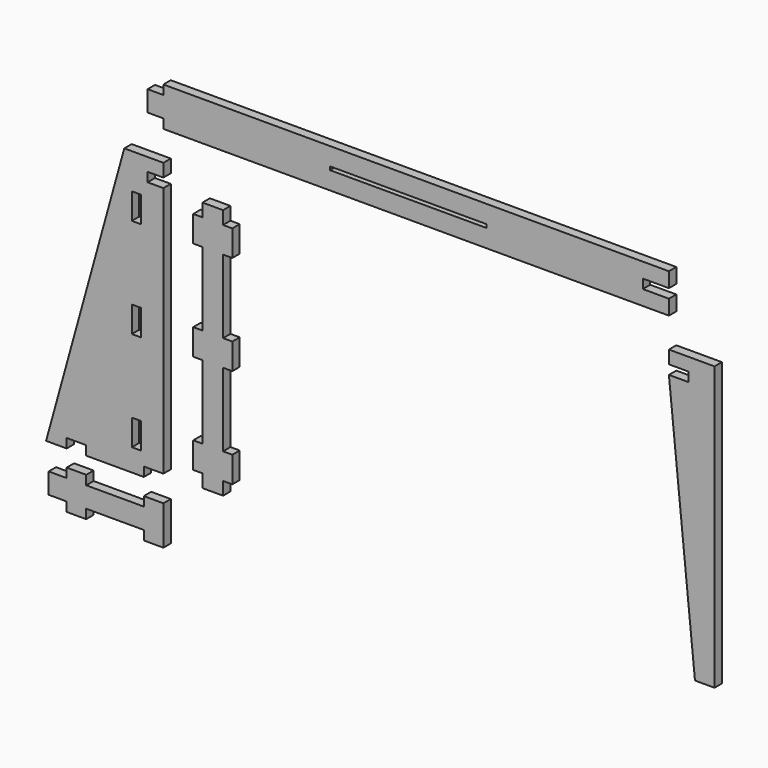
from build123d import *

# Parameters (mm, degrees)
F1_W     = 304.8
F1_H     = 6.604
F2_DEPTH = 18.034
F1_W_2   = 18.034
F1_H_2   = 50.8
F1_W_3   = 38.1
F1_H_3   = 18.034


# Not quite as in the source:
# - a variable given as a bare number and used for a length is read in inches; the dataset says mm whatever the document's units were


with BuildPart() as f2:
    # F1 (on Front) → F2 (new body)
    with BuildSketch(Plane.XZ):
        Polygon((508, 0), (-477.266, 0), (-477.266, -18.034), (-508, -18.034), (-508, -58.166), (-477.266, -58.166), (-477.266, -76.2), (508, -76.2), (508, -47.117), (457.2, -47.117), (457.2, -29.083), (508, -29.083), align=None)
        with Locations((0, -38.1)):
            Rectangle(F1_W, F1_H, mode=Mode.SUBTRACT)
    extrude(amount=F2_DEPTH)


with BuildPart() as f2b:
    # F1 (on Front) → F2, piece 2 (new body)
    with BuildSketch(Plane.XZ):
        Polygon((596.9, -685.8), (596.9, -134.366), (508, -134.366), (508, -159.766), (546.1, -159.766), (546.1, -177.8), (508, -177.8), (558.8, -685.8), align=None)
    extrude(amount=F2_DEPTH)


with BuildPart() as f2c:
    # F1 (on Front) → F2, piece 3 (new body)
    with BuildSketch(Plane.XZ):
        Polygon((-477.266, -667.766), (-477.266, -177.8), (-508, -177.8), (-508, -159.766), (-477.266, -159.766), (-477.266, -134.366), (-553.466, -134.366), (-705.866, -685.8), (-665.734, -685.8), (-665.734, -667.766), (-627.634, -667.766), (-627.634, -685.8), (-515.366, -685.8), (-515.366, -667.766), align=None)
        with Locations((-529.717, -616.966)):
            Rectangle(F1_W_2, F1_H_2, mode=Mode.SUBTRACT)
        with Locations((-529.717, -422.783)):
            Rectangle(F1_W_2, F1_H_2, mode=Mode.SUBTRACT)
        with Locations((-529.717, -228.6)):
            Rectangle(F1_W_2, F1_H_2, mode=Mode.SUBTRACT)
    extrude(amount=F2_DEPTH)


with BuildPart() as f2d:
    # F1 (on Front) → F2, piece 4 (new body)
    with BuildSketch(Plane.XZ):
        with Locations((-410.083, -228.6)):
            Rectangle(F1_W_2, F1_H_2)
        with Locations((-351.917, -228.6)):
            Rectangle(F1_W_2, F1_H_2)
        with Locations((-351.917, -422.783)):
            Rectangle(F1_W_2, F1_H_2)
        with Locations((-410.083, -422.783)):
            Rectangle(F1_W_2, F1_H_2)
        with Locations((-410.083, -616.966)):
            Rectangle(F1_W_2, F1_H_2)
        with Locations((-351.917, -616.966)):
            Rectangle(F1_W_2, F1_H_2)
        Polygon((-360.934, -177.8), (-401.066, -177.8), (-401.066, -203.2), (-401.066, -254), (-401.066, -397.383), (-401.066, -448.183), (-401.066, -591.566), (-401.066, -642.366), (-401.066, -667.766), (-360.934, -667.766), (-360.934, -642.366), (-360.934, -591.566), (-360.934, -448.183), (-360.934, -397.383), (-360.934, -254), (-360.934, -203.2), align=None)
    extrude(amount=F2_DEPTH)


with BuildPart() as f2e:
    # F1 (on Front) → F2, piece 5 (new body)
    with BuildSketch(Plane.XZ):
        with Locations((-496.316, -727.583)):
            Rectangle(F1_W_3, F1_H_3)
        Polygon((-665.734, -736.6), (-700.8819373561, -736.6), (-700.8819373561, -776.732), (-665.734, -776.732), (-627.634, -776.732), (-515.366, -776.732), (-477.266, -776.732), (-477.266, -736.6), (-515.366, -736.6), (-627.634, -736.6), align=None)
        with Locations((-496.316, -785.749)):
            Rectangle(F1_W_3, F1_H_3)
        with Locations((-646.684, -727.583)):
            Rectangle(F1_W_3, F1_H_3)
        with Locations((-646.684, -785.749)):
            Rectangle(F1_W_3, F1_H_3)
    extrude(amount=F2_DEPTH)


solid = Compound([f2.part, f2b.part, f2c.part, f2d.part, f2e.part])
